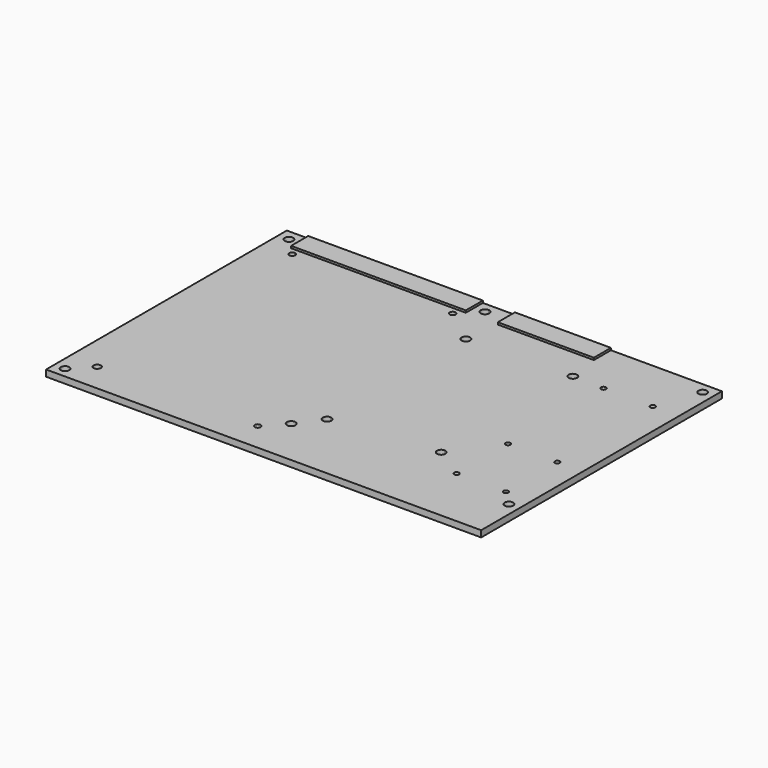
from build123d import *

# Parameters (mm, degrees)
F0_W     = 15
F0_H     = 10
F1_DEPTH = 3
F2_DEPTH = 4
F3_DEPTH = 4


# Not quite as in the source:
# - a feature names something its author has since deleted; it is built from what else it names


with BuildPart() as f1:
    # F0 (on Top) → F1 (new body)
    with BuildSketch(Plane.XY):
        with BuildLine():
            Line((-139.3440142274, -114.756315279), (-139.3440142274, -14.656315279))
            Line((-139.3440142274, -14.656315279), (-141.3440142274, -14.656315279))
            ThreePointArc((-141.3440142274, -14.656315279), (-143.7339637211, -15.6462647727), (-142.7440142274, -13.256315279))
            Line((-142.7440142274, -13.256315279), (-142.7440142274, -11.256315279))
            Line((-142.7440142274, -11.256315279), (-217.9440142274, -11.256315279))
            Line((-217.9440142274, -11.256315279), (-217.9440142274, -13.256315279))
            ThreePointArc((-217.9440142274, -13.256315279), (-216.9540647337, -13.6663657853), (-216.5440142274, -14.656315279))
            ThreePointArc((-216.5440142274, -14.656315279), (-217.9440142274, -16.056315279), (-219.3440142274, -14.656315279))
            Line((-219.3440142274, -14.656315279), (-221.1930548072, -14.656315279))
            Line((-221.1930548072, -14.656315279), (-221.1930548072, -128.856315279))
            Line((-221.1930548072, -128.856315279), (-219.6440142274, -128.856315279))
            ThreePointArc((-219.6440142274, -128.856315279), (-217.9440142274, -127.156315279), (-216.2440142274, -128.856315279))
            ThreePointArc((-216.2440142274, -128.856315279), (-216.7419326994, -130.058396807), (-217.9440142274, -130.556315279))
            Line((-217.9440142274, -130.556315279), (-217.9440142274, -132.256315279))
            Line((-217.9440142274, -132.256315279), (-142.7440142274, -132.256315279))
            Line((-142.7440142274, -132.256315279), (-142.7440142274, -130.256315279))
            ThreePointArc((-142.7440142274, -130.256315279), (-143.7339637211, -127.8663657853), (-141.3440142274, -128.856315279))
            Line((-141.3440142274, -128.856315279), (-139.3440142274, -128.856315279))
            Line((-139.3440142274, -128.856315279), (-139.3440142274, -124.756315279))
            Line((-139.3440142274, -124.756315279), (-139.3440142274, -119.756315279))
            Line((-139.3440142274, -119.756315279), (-139.3440142274, -114.756315279))
        make_face()
        with BuildLine():
            Line((-126.5440142274, -11.256315279), (-129.3440142274, -11.256315279))
            Line((-129.3440142274, -11.256315279), (-129.3440142274, -14.056315279))
            Line((-129.3440142274, -14.056315279), (-129.3440142274, -27.456315279))
            Line((-129.3440142274, -27.456315279), (-128.3440142274, -27.456315279))
            ThreePointArc((-128.3440142274, -27.456315279), (-126.3440142274, -25.456315279), (-124.3440142274, -27.456315279))
            ThreePointArc((-124.3440142274, -27.456315279), (-124.929800665, -28.8705288414), (-126.3440142274, -29.456315279))
            Line((-126.3440142274, -29.456315279), (-126.3440142274, -106.756315279))
            ThreePointArc((-126.3440142274, -106.756315279), (-124.929800665, -107.3421017166), (-124.3440142274, -108.756315279))
            ThreePointArc((-124.3440142274, -108.756315279), (-124.929800665, -110.1705288414), (-126.3440142274, -110.756315279))
            Line((-126.3440142274, -110.756315279), (-126.3440142274, -114.756315279))
            Line((-126.3440142274, -114.756315279), (-77.3440142274, -114.756315279))
            Line((-77.3440142274, -114.756315279), (-77.3440142274, -105.156315279))
            ThreePointArc((-77.3440142274, -105.156315279), (-79.3440142274, -103.156315279), (-77.3440142274, -101.156315279))
            Line((-77.3440142274, -101.156315279), (-77.3440142274, -28.056315279))
            ThreePointArc((-77.3440142274, -28.056315279), (-78.7582277898, -24.6421017166), (-75.3440142274, -26.056315279))
            Line((-75.3440142274, -26.056315279), (-74.3440142274, -26.056315279))
            Line((-74.3440142274, -26.056315279), (-74.3440142274, -14.256315279))
            Line((-74.3440142274, -14.256315279), (-74.3440142274, -11.256315279))
            Line((-74.3440142274, -11.256315279), (-77.3440142274, -11.256315279))
            Line((-77.3440142274, -11.256315279), (-79.3440142274, -11.256315279))
            Line((-79.3440142274, -11.256315279), (-124.3440142274, -11.256315279))
            Line((-124.3440142274, -11.256315279), (-126.3440142274, -11.256315279))
            Line((-126.3440142274, -11.256315279), (-126.5440142274, -11.256315279))
        make_face()
        Polygon((-32.3440142274, -11.256315279), (-74.3440142274, -11.256315279), (-74.3440142274, -14.256315279), (-74.3440142274, -26.056315279), (-74.3440142274, -103.156315279), (-74.3440142274, -111.906315279), (-74.3440142274, -114.756315279), (-64.3440142274, -114.756315279), (-64.3440142274, -112.806315279), (-64.3440142274, -82.706315279), (-64.3440142274, -80.756315279), (-62.3940142274, -80.756315279), (-57.3440142274, -80.756315279), (-57.3440142274, -70.756315279), (-42.3440142274, -70.756315279), (-42.3440142274, -80.756315279), (-39.2940142274, -80.756315279), (-37.3440142274, -80.756315279), (-37.3440142274, -82.706315279), (-37.3440142274, -112.806315279), (-37.3440142274, -114.756315279), (-27.3440142274, -114.756315279), (-27.3440142274, -14.656315279), (-27.3440142274, -11.256315279), align=None)
        Polygon((-62.5940142274, -60.756315279), (-64.3440142274, -60.756315279), (-64.3440142274, -59.006315279), (-64.3440142274, -26.456315279), (-64.3440142274, -24.756315279), (-62.6440142274, -24.756315279), (-39.5440142274, -24.756315279), (-37.8440142274, -24.756315279), (-37.8440142274, -26.456315279), (-37.8440142274, -59.006315279), (-37.8440142274, -60.756315279), (-39.5940142274, -60.756315279), align=None, mode=Mode.SUBTRACT)
        Polygon((-37.3440142274, -124.756315279), (-129.3440142274, -124.756315279), (-129.3440142274, -142.256315279), (-27.3440142274, -142.256315279), (-27.3440142274, -124.756315279), (-32.3440142274, -124.756315279), align=None)
        with BuildLine():
            Line((-221.1930548072, -6.256315279), (-221.1930548072, -1.256315279))
            Line((-221.1930548072, -1.256315279), (-231.1930548072, -1.256315279))
            Line((-231.1930548072, -1.256315279), (-231.1930548072, -132.256315279))
            Line((-231.1930548072, -132.256315279), (-221.1930548072, -132.256315279))
            Line((-221.1930548072, -132.256315279), (-221.1930548072, -128.856315279))
            Line((-221.1930548072, -128.856315279), (-221.1930548072, -14.656315279))
            Line((-221.1930548072, -14.656315279), (-221.1930548072, -11.256315279))
            Line((-221.1930548072, -11.256315279), (-226.1930548072, -11.256315279))
            Line((-226.1930548072, -11.256315279), (-226.1930548072, -8.256315279))
            ThreePointArc((-226.1930548072, -8.256315279), (-227.6072683696, -4.8421017166), (-224.1930548072, -6.256315279))
            Line((-224.1930548072, -6.256315279), (-221.1930548072, -6.256315279))
        make_face()
        Polygon((-139.1930548072, -11.256315279), (-139.3440142274, -11.256315279), (-139.3440142274, -14.656315279), (-139.3440142274, -114.756315279), (-129.3440142274, -114.756315279), (-129.3440142274, -111.756315279), (-129.3440142274, -108.756315279), (-129.3440142274, -27.956315279), (-129.3440142274, -27.456315279), (-129.3440142274, -14.056315279), (-129.3440142274, -11.256315279), align=None)
        with BuildLine():
            Line((-64.3440142274, -59.006315279), (-64.3440142274, -60.756315279))
            Line((-64.3440142274, -60.756315279), (-62.5940142274, -60.756315279))
            Line((-62.5940142274, -60.756315279), (-39.5940142274, -60.756315279))
            Line((-39.5940142274, -60.756315279), (-37.8440142274, -60.756315279))
            Line((-37.8440142274, -60.756315279), (-37.8440142274, -59.006315279))
            Line((-37.8440142274, -59.006315279), (-37.8440142274, -26.456315279))
            Line((-37.8440142274, -26.456315279), (-38.3440142274, -26.456315279))
            ThreePointArc((-38.3440142274, -26.456315279), (-40.3925423648, -27.3048434164), (-39.5440142274, -25.256315279))
            Line((-39.5440142274, -25.256315279), (-39.5440142274, -24.756315279))
            Line((-39.5440142274, -24.756315279), (-62.6440142274, -24.756315279))
            Line((-62.6440142274, -24.756315279), (-62.6440142274, -25.256315279))
            ThreePointArc((-62.6440142274, -25.256315279), (-61.79548609, -25.6077871416), (-61.4440142274, -26.456315279))
            ThreePointArc((-61.4440142274, -26.456315279), (-62.6440142274, -27.656315279), (-63.8440142274, -26.456315279))
            Line((-63.8440142274, -26.456315279), (-64.3440142274, -26.456315279))
            Line((-64.3440142274, -26.456315279), (-64.3440142274, -59.006315279))
        make_face()
        Polygon((-126.3440142274, -114.756315279), (-129.3440142274, -114.756315279), (-129.3440142274, -124.756315279), (-37.3440142274, -124.756315279), (-37.3440142274, -119.756315279), (-37.3440142274, -114.756315279), (-39.2940142274, -114.756315279), (-62.3940142274, -114.756315279), (-64.3440142274, -114.756315279), (-74.3440142274, -114.756315279), (-77.1940142274, -114.756315279), (-77.3440142274, -114.756315279), align=None)
        with BuildLine():
            Line((-62.3940142274, -114.756315279), (-39.2940142274, -114.756315279))
            Line((-39.2940142274, -114.756315279), (-39.2940142274, -113.956315279))
            ThreePointArc((-39.2940142274, -113.956315279), (-40.1071870258, -111.9931424806), (-38.1440142274, -112.806315279))
            Line((-38.1440142274, -112.806315279), (-37.3440142274, -112.806315279))
            Line((-37.3440142274, -112.806315279), (-37.3440142274, -82.706315279))
            Line((-37.3440142274, -82.706315279), (-38.1440142274, -82.706315279))
            ThreePointArc((-38.1440142274, -82.706315279), (-40.1071870258, -83.5194880774), (-39.2940142274, -81.556315279))
            Line((-39.2940142274, -81.556315279), (-39.2940142274, -80.756315279))
            Line((-39.2940142274, -80.756315279), (-42.3440142274, -80.756315279))
            Line((-42.3440142274, -80.756315279), (-57.3440142274, -80.756315279))
            Line((-57.3440142274, -80.756315279), (-62.3940142274, -80.756315279))
            Line((-62.3940142274, -80.756315279), (-62.3940142274, -81.556315279))
            ThreePointArc((-62.3940142274, -81.556315279), (-61.580841429, -81.8931424806), (-61.2440142274, -82.706315279))
            ThreePointArc((-61.2440142274, -82.706315279), (-62.3940142274, -83.856315279), (-63.5440142274, -82.706315279))
            Line((-63.5440142274, -82.706315279), (-64.3440142274, -82.706315279))
            Line((-64.3440142274, -82.706315279), (-64.3440142274, -112.806315279))
            Line((-64.3440142274, -112.806315279), (-63.5440142274, -112.806315279))
            ThreePointArc((-63.5440142274, -112.806315279), (-62.3940142274, -111.656315279), (-61.2440142274, -112.806315279))
            ThreePointArc((-61.2440142274, -112.806315279), (-61.580841429, -113.6194880774), (-62.3940142274, -113.956315279))
            Line((-62.3940142274, -113.956315279), (-62.3940142274, -114.756315279))
        make_face()
        Polygon((-217.9440142274, -132.256315279), (-221.1930548072, -132.256315279), (-221.1930548072, -142.256315279), (-139.1930548072, -142.256315279), (-139.3440142274, -132.256315279), (-142.7440142274, -132.256315279), align=None)
        Polygon((-139.3440142274, -6.256315279), (-139.3440142274, -1.256315279), (-221.1930548072, -1.256315279), (-221.1930548072, -6.256315279), (-221.1930548072, -11.256315279), (-217.9440142274, -11.256315279), (-142.7440142274, -11.256315279), (-139.3440142274, -11.256315279), align=None)
        with BuildLine():
            Line((-79.3440142274, -1.256315279), (-79.3440142274, -11.256315279))
            Line((-79.3440142274, -11.256315279), (-77.3440142274, -11.256315279))
            Line((-77.3440142274, -11.256315279), (-74.3440142274, -11.256315279))
            Line((-74.3440142274, -11.256315279), (-32.3440142274, -11.256315279))
            Line((-32.3440142274, -11.256315279), (-32.3440142274, -8.256315279))
            ThreePointArc((-32.3440142274, -8.256315279), (-33.7582277898, -4.8421017166), (-30.3440142274, -6.256315279))
            Line((-30.3440142274, -6.256315279), (-27.3440142274, -6.256315279))
            Line((-27.3440142274, -6.256315279), (-27.3440142274, -1.256315279))
            Line((-27.3440142274, -1.256315279), (-79.3440142274, -1.256315279))
        make_face()
        Polygon((-83.3440142274, -1.256315279), (-124.3440142274, -1.256315279), (-124.3440142274, -11.256315279), (-79.3440142274, -11.256315279), (-79.3440142274, -1.256315279), align=None)
        with BuildLine():
            Line((-128.3440142274, -27.456315279), (-129.3440142274, -27.456315279))
            Line((-129.3440142274, -27.456315279), (-129.3440142274, -27.956315279))
            Line((-129.3440142274, -27.956315279), (-129.3440142274, -108.756315279))
            Line((-129.3440142274, -108.756315279), (-128.3440142274, -108.756315279))
            ThreePointArc((-128.3440142274, -108.756315279), (-127.7582277898, -107.3421017166), (-126.3440142274, -106.756315279))
            Line((-126.3440142274, -106.756315279), (-126.3440142274, -29.456315279))
            ThreePointArc((-126.3440142274, -29.456315279), (-127.7582277898, -28.8705288414), (-128.3440142274, -27.456315279))
        make_face()
        with BuildLine():
            Line((-74.3440142274, -103.156315279), (-74.3440142274, -26.056315279))
            Line((-74.3440142274, -26.056315279), (-75.3440142274, -26.056315279))
            ThreePointArc((-75.3440142274, -26.056315279), (-75.929800665, -27.4705288414), (-77.3440142274, -28.056315279))
            Line((-77.3440142274, -28.056315279), (-77.3440142274, -101.156315279))
            ThreePointArc((-77.3440142274, -101.156315279), (-75.929800665, -101.7421017166), (-75.3440142274, -103.156315279))
            Line((-75.3440142274, -103.156315279), (-74.3440142274, -103.156315279))
        make_face()
        Polygon((-129.3440142274, -142.256315279), (-129.3440142274, -124.756315279), (-134.3440142274, -124.756315279), (-139.1930548072, -124.756315279), (-139.3440142274, -124.756315279), (-139.3440142274, -128.856315279), (-139.3440142274, -132.256315279), (-139.1930548072, -142.256315279), align=None)
        with Locations((-49.8440142274, -75.756315279)):
            Rectangle(F0_W, F0_H)
        with BuildLine():
            Line((-221.1930548072, -132.256315279), (-231.1930548072, -132.256315279))
            Line((-231.1930548072, -132.256315279), (-231.1930548072, -137.3912245035))
            Line((-231.1930548072, -137.3912245035), (-228.1930548072, -137.3912245035))
            ThreePointArc((-228.1930548072, -137.3912245035), (-226.1930548072, -135.3912245035), (-224.1930548072, -137.3912245035))
            ThreePointArc((-224.1930548072, -137.3912245035), (-224.7788412448, -138.8054380659), (-226.1930548072, -139.3912245035))
            Line((-226.1930548072, -139.3912245035), (-226.1930548072, -142.256315279))
            Line((-226.1930548072, -142.256315279), (-221.1930548072, -142.256315279))
            Line((-221.1930548072, -142.256315279), (-221.1930548072, -132.256315279))
        make_face()
        with BuildLine():
            Line((-129.3440142274, -1.256315279), (-134.3440142274, -1.256315279))
            Line((-134.3440142274, -1.256315279), (-134.3440142274, -4.256315279))
            ThreePointArc((-134.3440142274, -4.256315279), (-132.929800665, -4.8421017166), (-132.3440142274, -6.256315279))
            ThreePointArc((-132.3440142274, -6.256315279), (-134.3440142274, -8.256315279), (-136.3440142274, -6.256315279))
            Line((-136.3440142274, -6.256315279), (-139.3440142274, -6.256315279))
            Line((-139.3440142274, -6.256315279), (-139.3440142274, -11.256315279))
            Line((-139.3440142274, -11.256315279), (-139.1930548072, -11.256315279))
            Line((-139.1930548072, -11.256315279), (-129.3440142274, -11.256315279))
            Line((-129.3440142274, -11.256315279), (-129.3440142274, -1.256315279))
        make_face()
        with BuildLine():
            Line((-129.3440142274, -114.756315279), (-139.3440142274, -114.756315279))
            Line((-139.3440142274, -114.756315279), (-139.3440142274, -119.756315279))
            Line((-139.3440142274, -119.756315279), (-136.3440142274, -119.756315279))
            ThreePointArc((-136.3440142274, -119.756315279), (-134.3440142274, -117.756315279), (-132.3440142274, -119.756315279))
            ThreePointArc((-132.3440142274, -119.756315279), (-132.929800665, -121.1705288414), (-134.3440142274, -121.756315279))
            Line((-134.3440142274, -121.756315279), (-134.3440142274, -124.756315279))
            Line((-134.3440142274, -124.756315279), (-129.3440142274, -124.756315279))
            Line((-129.3440142274, -124.756315279), (-129.3440142274, -114.756315279))
        make_face()
        with BuildLine():
            Line((-32.3440142274, -121.756315279), (-32.3440142274, -124.756315279))
            Line((-32.3440142274, -124.756315279), (-27.3440142274, -124.756315279))
            Line((-27.3440142274, -124.756315279), (-27.3440142274, -114.756315279))
            Line((-27.3440142274, -114.756315279), (-37.3440142274, -114.756315279))
            Line((-37.3440142274, -114.756315279), (-37.3440142274, -119.756315279))
            Line((-37.3440142274, -119.756315279), (-34.3440142274, -119.756315279))
            ThreePointArc((-34.3440142274, -119.756315279), (-32.3440142274, -117.756315279), (-30.3440142274, -119.756315279))
            ThreePointArc((-30.3440142274, -119.756315279), (-30.929800665, -121.1705288414), (-32.3440142274, -121.756315279))
        make_face()
        Polygon((-124.3440142274, -1.256315279), (-129.3440142274, -1.256315279), (-129.3440142274, -11.256315279), (-126.5440142274, -11.256315279), (-126.3440142274, -11.256315279), (-124.3440142274, -11.256315279), align=None)
        with BuildLine():
            Line((-77.3440142274, -105.156315279), (-77.3440142274, -114.756315279))
            Line((-77.3440142274, -114.756315279), (-77.1940142274, -114.756315279))
            Line((-77.1940142274, -114.756315279), (-74.3440142274, -114.756315279))
            Line((-74.3440142274, -114.756315279), (-74.3440142274, -111.906315279))
            Line((-74.3440142274, -111.906315279), (-74.3440142274, -103.156315279))
            Line((-74.3440142274, -103.156315279), (-75.3440142274, -103.156315279))
            ThreePointArc((-75.3440142274, -103.156315279), (-75.929800665, -104.5705288414), (-77.3440142274, -105.156315279))
        make_face()
        with BuildLine():
            Line((-134.3440142274, -1.256315279), (-139.3440142274, -1.256315279))
            Line((-139.3440142274, -1.256315279), (-139.3440142274, -6.256315279))
            Line((-139.3440142274, -6.256315279), (-136.3440142274, -6.256315279))
            ThreePointArc((-136.3440142274, -6.256315279), (-135.7582277898, -4.8421017166), (-134.3440142274, -4.256315279))
            Line((-134.3440142274, -4.256315279), (-134.3440142274, -1.256315279))
        make_face()
        with BuildLine():
            Line((-221.1930548072, -11.256315279), (-221.1930548072, -6.256315279))
            Line((-221.1930548072, -6.256315279), (-224.1930548072, -6.256315279))
            ThreePointArc((-224.1930548072, -6.256315279), (-224.7788412448, -7.6705288414), (-226.1930548072, -8.256315279))
            Line((-226.1930548072, -8.256315279), (-226.1930548072, -11.256315279))
            Line((-226.1930548072, -11.256315279), (-221.1930548072, -11.256315279))
        make_face()
        with BuildLine():
            Line((-136.3440142274, -119.756315279), (-139.3440142274, -119.756315279))
            Line((-139.3440142274, -119.756315279), (-139.3440142274, -124.756315279))
            Line((-139.3440142274, -124.756315279), (-139.1930548072, -124.756315279))
            Line((-139.1930548072, -124.756315279), (-134.3440142274, -124.756315279))
            Line((-134.3440142274, -124.756315279), (-134.3440142274, -121.756315279))
            ThreePointArc((-134.3440142274, -121.756315279), (-135.7582277898, -121.1705288414), (-136.3440142274, -119.756315279))
        make_face()
        with BuildLine():
            Line((-27.3440142274, -11.256315279), (-27.3440142274, -6.256315279))
            Line((-27.3440142274, -6.256315279), (-30.3440142274, -6.256315279))
            ThreePointArc((-30.3440142274, -6.256315279), (-30.929800665, -7.6705288414), (-32.3440142274, -8.256315279))
            Line((-32.3440142274, -8.256315279), (-32.3440142274, -11.256315279))
            Line((-32.3440142274, -11.256315279), (-27.3440142274, -11.256315279))
        make_face()
        with BuildLine():
            Line((-37.3440142274, -119.756315279), (-37.3440142274, -124.756315279))
            Line((-37.3440142274, -124.756315279), (-32.3440142274, -124.756315279))
            Line((-32.3440142274, -124.756315279), (-32.3440142274, -121.756315279))
            ThreePointArc((-32.3440142274, -121.756315279), (-33.7582277898, -121.1705288414), (-34.3440142274, -119.756315279))
            Line((-34.3440142274, -119.756315279), (-37.3440142274, -119.756315279))
        make_face()
        with BuildLine():
            Line((-228.1930548072, -137.3912245035), (-231.1930548072, -137.3912245035))
            Line((-231.1930548072, -137.3912245035), (-231.1930548072, -142.256315279))
            Line((-231.1930548072, -142.256315279), (-226.1930548072, -142.256315279))
            Line((-226.1930548072, -142.256315279), (-226.1930548072, -139.3912245035))
            ThreePointArc((-226.1930548072, -139.3912245035), (-227.6072683696, -138.8054380659), (-228.1930548072, -137.3912245035))
        make_face()
        with BuildLine():
            Line((-129.3440142274, -111.756315279), (-129.3440142274, -114.756315279))
            Line((-129.3440142274, -114.756315279), (-126.3440142274, -114.756315279))
            Line((-126.3440142274, -114.756315279), (-126.3440142274, -110.756315279))
            ThreePointArc((-126.3440142274, -110.756315279), (-127.7582277898, -110.1705288414), (-128.3440142274, -108.756315279))
            Line((-128.3440142274, -108.756315279), (-129.3440142274, -108.756315279))
            Line((-129.3440142274, -108.756315279), (-129.3440142274, -111.756315279))
        make_face()
        with BuildLine():
            Line((-139.3440142274, -14.656315279), (-139.3440142274, -11.256315279))
            Line((-139.3440142274, -11.256315279), (-142.7440142274, -11.256315279))
            Line((-142.7440142274, -11.256315279), (-142.7440142274, -13.256315279))
            ThreePointArc((-142.7440142274, -13.256315279), (-141.7540647337, -13.6663657853), (-141.3440142274, -14.656315279))
            Line((-141.3440142274, -14.656315279), (-139.3440142274, -14.656315279))
        make_face()
        with BuildLine():
            Line((-142.7440142274, -130.256315279), (-142.7440142274, -132.256315279))
            Line((-142.7440142274, -132.256315279), (-139.3440142274, -132.256315279))
            Line((-139.3440142274, -132.256315279), (-139.3440142274, -128.856315279))
            Line((-139.3440142274, -128.856315279), (-141.3440142274, -128.856315279))
            ThreePointArc((-141.3440142274, -128.856315279), (-141.7540647337, -129.8462647727), (-142.7440142274, -130.256315279))
        make_face()
        with BuildLine():
            Line((-217.9440142274, -11.256315279), (-221.1930548072, -11.256315279))
            Line((-221.1930548072, -11.256315279), (-221.1930548072, -14.656315279))
            Line((-221.1930548072, -14.656315279), (-219.3440142274, -14.656315279))
            ThreePointArc((-219.3440142274, -14.656315279), (-218.9339637211, -13.6663657853), (-217.9440142274, -13.256315279))
            Line((-217.9440142274, -13.256315279), (-217.9440142274, -11.256315279))
        make_face()
        with BuildLine():
            Line((-221.1930548072, -128.856315279), (-221.1930548072, -132.256315279))
            Line((-221.1930548072, -132.256315279), (-217.9440142274, -132.256315279))
            Line((-217.9440142274, -132.256315279), (-217.9440142274, -130.556315279))
            ThreePointArc((-217.9440142274, -130.556315279), (-219.1460957554, -130.058396807), (-219.6440142274, -128.856315279))
            Line((-219.6440142274, -128.856315279), (-221.1930548072, -128.856315279))
        make_face()
        with BuildLine():
            Line((-39.2940142274, -114.756315279), (-37.3440142274, -114.756315279))
            Line((-37.3440142274, -114.756315279), (-37.3440142274, -112.806315279))
            Line((-37.3440142274, -112.806315279), (-38.1440142274, -112.806315279))
            ThreePointArc((-38.1440142274, -112.806315279), (-38.480841429, -113.6194880774), (-39.2940142274, -113.956315279))
            Line((-39.2940142274, -113.956315279), (-39.2940142274, -114.756315279))
        make_face()
        with BuildLine():
            Line((-64.3440142274, -112.806315279), (-64.3440142274, -114.756315279))
            Line((-64.3440142274, -114.756315279), (-62.3940142274, -114.756315279))
            Line((-62.3940142274, -114.756315279), (-62.3940142274, -113.956315279))
            ThreePointArc((-62.3940142274, -113.956315279), (-63.2071870258, -113.6194880774), (-63.5440142274, -112.806315279))
            Line((-63.5440142274, -112.806315279), (-64.3440142274, -112.806315279))
        make_face()
        with BuildLine():
            Line((-38.1440142274, -82.706315279), (-37.3440142274, -82.706315279))
            Line((-37.3440142274, -82.706315279), (-37.3440142274, -80.756315279))
            Line((-37.3440142274, -80.756315279), (-39.2940142274, -80.756315279))
            Line((-39.2940142274, -80.756315279), (-39.2940142274, -81.556315279))
            ThreePointArc((-39.2940142274, -81.556315279), (-38.480841429, -81.8931424806), (-38.1440142274, -82.706315279))
        make_face()
        with BuildLine():
            Line((-64.3440142274, -80.756315279), (-64.3440142274, -82.706315279))
            Line((-64.3440142274, -82.706315279), (-63.5440142274, -82.706315279))
            ThreePointArc((-63.5440142274, -82.706315279), (-63.2071870258, -81.8931424806), (-62.3940142274, -81.556315279))
            Line((-62.3940142274, -81.556315279), (-62.3940142274, -80.756315279))
            Line((-62.3940142274, -80.756315279), (-64.3440142274, -80.756315279))
        make_face()
        with BuildLine():
            Line((-64.3440142274, -24.756315279), (-64.3440142274, -26.456315279))
            Line((-64.3440142274, -26.456315279), (-63.8440142274, -26.456315279))
            ThreePointArc((-63.8440142274, -26.456315279), (-63.4925423648, -25.6077871416), (-62.6440142274, -25.256315279))
            Line((-62.6440142274, -25.256315279), (-62.6440142274, -24.756315279))
            Line((-62.6440142274, -24.756315279), (-64.3440142274, -24.756315279))
        make_face()
        with BuildLine():
            Line((-38.3440142274, -26.456315279), (-37.8440142274, -26.456315279))
            Line((-37.8440142274, -26.456315279), (-37.8440142274, -24.756315279))
            Line((-37.8440142274, -24.756315279), (-39.5440142274, -24.756315279))
            Line((-39.5440142274, -24.756315279), (-39.5440142274, -25.256315279))
            ThreePointArc((-39.5440142274, -25.256315279), (-38.69548609, -25.6077871416), (-38.3440142274, -26.456315279))
        make_face()
    extrude(amount=F1_DEPTH)

    # F0 (on Top) → F2 (join)
    with BuildSketch(Plane.XY):
        Polygon((-139.3440142274, -6.256315279), (-139.3440142274, -1.256315279), (-221.1930548072, -1.256315279), (-221.1930548072, -6.256315279), (-221.1930548072, -11.256315279), (-217.9440142274, -11.256315279), (-142.7440142274, -11.256315279), (-139.3440142274, -11.256315279), align=None)
    extrude(amount=F2_DEPTH)

    # F0 (on Top) → F3 (join)
    with BuildSketch(Plane.XY):
        Polygon((-83.3440142274, -1.256315279), (-124.3440142274, -1.256315279), (-124.3440142274, -11.256315279), (-79.3440142274, -11.256315279), (-79.3440142274, -1.256315279), align=None)
    extrude(amount=F3_DEPTH)


solid = f1.part
